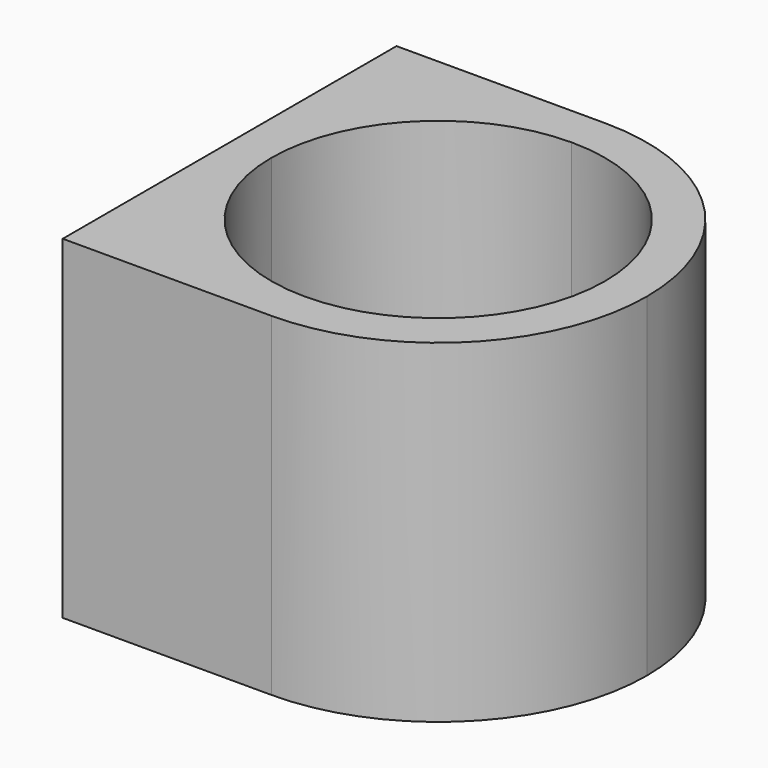
from build123d import *

# Parameters (mm, degrees)
F1_DEPTH = 25.4
F2_R     = 12.7
F3_DEPTH = 3.175
F5_DEPTH = 12.7


with BuildPart() as f1:
    # F0 (on Top) → F1 (new body)
    with BuildSketch(Plane.XY):
        with BuildLine():
            ThreePointArc((-15.875, 0), (-11.2253201513, 11.2253201513), (0, 15.875))
            Line((0, 15.875), (-15.875, 15.875))
            Line((-15.875, 15.875), (-15.875, 0))
        make_face()
        with BuildLine():
            Line((-15.875, -15.875), (0, -15.875))
            ThreePointArc((0, -15.875), (-11.2253201513, -11.2253201513), (-15.875, 0))
            Line((-15.875, 0), (-15.875, -15.875))
        make_face()
        with BuildLine():
            Line((0, -15.875), (0, -12.7))
            ThreePointArc((0, -12.7), (-8.9802561211, -8.9802561211), (-12.7, 0))
            Line((-12.7, 0), (-15.875, 0))
            ThreePointArc((-15.875, 0), (-11.2253201513, -11.2253201513), (0, -15.875))
        make_face()
        with BuildLine():
            ThreePointArc((-12.7, 0), (-8.9802561211, 8.9802561211), (0, 12.7))
            Line((0, 12.7), (0, 15.875))
            ThreePointArc((0, 15.875), (-11.2253201513, 11.2253201513), (-15.875, 0))
            Line((-15.875, 0), (-12.7, 0))
        make_face()
        with BuildLine():
            ThreePointArc((0, 12.7), (8.9802561211, 8.9802561211), (12.7, 0))
            ThreePointArc((12.7, 0), (8.9802561211, -8.9802561211), (0, -12.7))
            Line((0, -12.7), (0, -15.875))
            ThreePointArc((0, -15.875), (11.2253201513, -11.2253201513), (15.875, 0))
            ThreePointArc((15.875, 0), (11.2253201513, 11.2253201513), (0, 15.875))
            Line((0, 15.875), (0, 12.7))
        make_face()
    extrude(amount=F1_DEPTH)

    # F2 (on face) → F3 (join)
    with BuildSketch(Plane(origin=(0, 0, 0), x_dir=(1, 0, 0), z_dir=(0, 0, -1))):
        with BuildLine():
            Line((-15.875, 15.875), (-15.875, -15.875))
            Line((-15.875, -15.875), (0, -15.875))
            ThreePointArc((0, -15.875), (15.875, 0), (0, 15.875))
            Line((0, 15.875), (-15.875, 15.875))
        make_face()
        Circle(F2_R, mode=Mode.SUBTRACT)
        Circle(F2_R)
    extrude(amount=-F3_DEPTH)

    # F4 (on face) → F5 (cut)
    with BuildSketch(Plane(origin=(-15.875, 0, 0), x_dir=(0, -1, 0), z_dir=(-1, 0, 0))):
        Polygon((0, 6.35), (0, 9.525), (-7.9375, 9.525), (-11.90625, 9.525), (-11.90625, 6.35), (-7.9375, 6.35), align=None)
        Polygon((7.9375, 9.525), (0, 9.525), (0, 6.35), (7.9375, 6.35), (11.90625, 6.35), (11.90625, 9.525), align=None)
    extrude(amount=-F5_DEPTH, mode=Mode.SUBTRACT)


solid = f1.part
